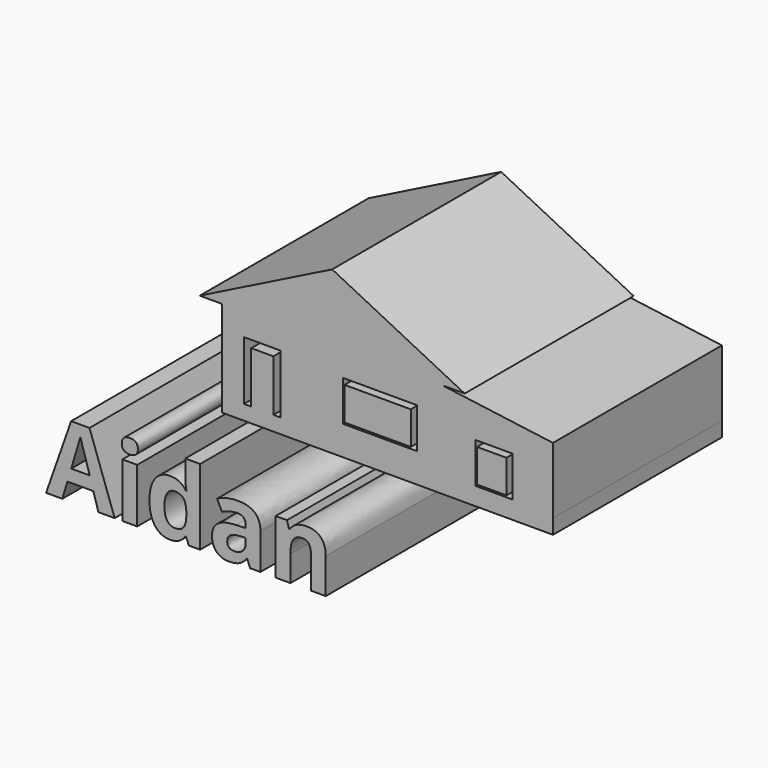
from build123d import *

# Parameters (mm, degrees)
F0_W         = 3048.0000034332
F0_H         = 1676.4000034332
F0_W_2       = 1524
F0_H_2       = 1676.4
F0_W_3       = 4572
F0_H_3       = 609.6
F0_TEXT_SIZE = 4116.3252459632
F1_DEPTH     = 8747.76
F2_W         = 1828.8
F2_H         = 1219.2
F3_DEPTH     = 60.96
F0_W_4       = 914.4
F0_H_4       = 2133.6
F4_DEPTH     = 8747.76
F0_W_5       = 2743.2
F0_H_5       = 1371.6
F5_DEPTH     = 30.48
F0_W_6       = 1219.2
F6_DEPTH     = 8839.2


# Not quite as in the source:
# - Text() gives the source's letters only with a copy of the font that has no kerning and outlines rounded to 1/6400 em; it was checked with that copy


with BuildPart() as f1:
    # F0 (on Front) → F1 (new body)
    with BuildSketch(Plane.XZ):
        Polygon((4572, 0), (0, 0), (-4572, 0), (-4572, -3352.8), (-3657.6, -3352.8), (-3657.6, -914.4), (-2133.6, -914.4), (-2133.6, -3352.8), (4572, -3352.8), (4572, -922.4951733378), align=None)
        with Locations((1981.2, -1905)):
            Rectangle(F0_W, F0_H, mode=Mode.SUBTRACT)
        Polygon((0, 2286), (0, 0), (4572, 0), align=None)
        Polygon((-4572, 0), (0, 0), (0, 2286), align=None)
        Polygon((-5486.4, 0), (-4572, 0), (0, 2286), (0, 2743.2), align=None)
        Polygon((0, 2286), (4572, 0), (5486.4, 0), (0, 2743.2), align=None)
        Polygon((9143.1556086981, -609.6001299571), (4572, 0), (4572, -922.4951733378), (9143.4395759312, -1532.1331725947), align=None)
        Polygon((-3657.6, -3352.8), (-4572, -3352.8), (-4572, -3962.4), (4572, -3962.4), (4572, -3352.8), (-2133.6, -3352.8), (-2438.4, -3352.8), (-3352.8, -3352.8), align=None)
        Polygon((9143.4395759312, -1532.1331725947), (4572, -922.4951733378), (4572, -3352.8), (9144, -3352.8), align=None)
        with Locations((6705.6, -2383.398846817)):
            Rectangle(F0_W_2, F0_H_2, mode=Mode.SUBTRACT)
        with Locations((6858, -3657.6)):
            Rectangle(F0_W_3, F0_H_3)
        with Locations((-11850.5144776363, -9258.2330703735)):
            Text('Aidan', F0_TEXT_SIZE, font='Open Sans', font_style=FontStyle.BOLD, text_align=(TextAlign.LEFT, TextAlign.BOTTOM))
    extrude(amount=F1_DEPTH)

    # F2 (on face) → F3 (join)
    with BuildSketch(Plane(origin=(-4572, 0, 0), x_dir=(0, -1, 0), z_dir=(-1, 0, 0))):
        with Locations((6386.12498703, -1371.6)):
            Rectangle(F2_W, F2_H)
        with Locations((2156.3082748413, -2683.608360672)):
            Rectangle(F2_W, F2_H)
    extrude(amount=F3_DEPTH)

    # F0 (on Front) → F4 (join)
    with BuildSketch(Plane.XZ):
        with Locations((-2895.6, -2286)):
            Rectangle(F0_W_4, F0_H_4)
    extrude(amount=F4_DEPTH)


with BuildPart() as f5:
    # F0 (on Front) → F5 (new body)
    with BuildSketch(Plane.XZ):
        with Locations((1981.2, -1905)):
            Rectangle(F0_W_5, F0_H_5)
    extrude(amount=F5_DEPTH)


with BuildPart() as f5b:
    # F0 (on Front) → F5, piece 2 (new body)
    with BuildSketch(Plane.XZ):
        with Locations((6705.6, -2383.398846817)):
            Rectangle(F0_W_6, F0_H_5)
    extrude(amount=F5_DEPTH)


with BuildPart() as f6:
    # F6 (new): a face of the model
    f6_faces = [f5.part.faces().sort_by_distance(p)[0] for p in [
        (1981.2, -30.48, -1905),
    ]]
    extrude(f6_faces, amount=F6_DEPTH)


with BuildPart() as f6b:
    # F6#2 (new): a face of the model
    f6_2_faces = [f5b.part.faces().sort_by_distance(p)[0] for p in [
        (6705.6, -30.48, -2383.398846817),
    ]]
    extrude(f6_2_faces, amount=F6_DEPTH)


solid = Compound([f1.part, f5.part, f5b.part, f6.part, f6b.part])
